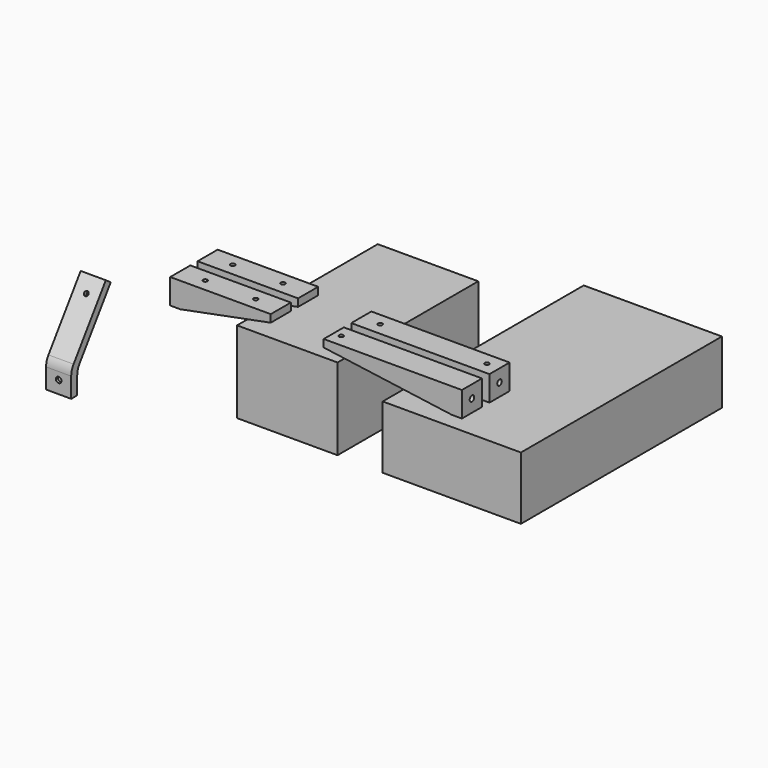
from build123d import *

# Parameters (mm, degrees)
F1_DEPTH   = 20
F3_R       = 1.75
F4_DEPTH   = 25
F5_R       = 3.5
F5_R_2     = 1.75
F6_DEPTH   = 3
F2_R       = 2.25
F7_DEPTH   = 25
F2_R_2     = 4
F8_DEPTH   = 4
F9_R       = 13
F10_W      = 80
F10_H      = 140
F11_DEPTH  = 65
F12_W      = 110
F12_H      = 200
F13_DEPTH  = 50
F15_DEPTH  = 20
F16_R      = 2.25
F17_DEPTH  = 122.8202211986
F18_DEPTH  = 4
F20_W      = 73.3484832836
F20_H      = 4
F22_R      = 1.75
F23_DEPTH  = 6.001
F22_R_2    = 3
F24_DEPTH  = 3
F26_DEPTH  = 20
F27_R      = 2.25
F28_DEPTH  = 4
F29_DEPTH  = 8.001
F31_W      = 102.9563014099
F31_H      = 4
F34_R      = 3
F34_R_2    = 1.75
F35_R      = 3
F35_R_2    = 1.75
F36_DEPTH  = 3
F36_FACE_R = 1.75
F37_DEPTH  = 9.6879868636
F38_DEPTH  = 3


with BuildPart() as f1:
    # F0 (on Right) → F1 (new body)
    with BuildSketch(Plane.YZ):
        Polygon((0, 20), (0, 0), (6, 0), (6, 18.1082072667), (39.3294984468, 65.7076640392), (34.4145861811, 69.1491226573), align=None)
    extrude(amount=F1_DEPTH)

    # F3 (on face) → F4 (cut)
    with BuildSketch(Plane(origin=(0, -9.3969262079, 6.5797985667), x_dir=(1, 0, 0), z_dir=(0, -0.8191520443, 0.5735764364))):
        with Locations((10, 64.3830408858)):
            Circle(F3_R)
    extrude(amount=-F4_DEPTH, mode=Mode.SUBTRACT)

    # F5 (on face) → F6 (cut)
    with BuildSketch(Plane(origin=(0, -4.4820139421, 3.1383399486), x_dir=(-1, 0, 0), z_dir=(0, 0.8191520443, -0.5735764364))):
        with Locations((-10, 64.3830408858)):
            Circle(F5_R)
        with Locations((-10, 64.3830408858)):
            Circle(F5_R_2, mode=Mode.SUBTRACT)
    extrude(amount=-F6_DEPTH, mode=Mode.SUBTRACT)

    # F2 (on face) → F7 (cut)
    with BuildSketch(Plane(origin=(0, 6, 0), x_dir=(-1, 0, 0), z_dir=(0, 1, 0))):
        with Locations((-10, 10)):
            Circle(F2_R)
    extrude(amount=-F7_DEPTH, mode=Mode.SUBTRACT)

    # F2 (on face) → F8 (cut)
    with BuildSketch(Plane(origin=(0, 6, 0), x_dir=(-1, 0, 0), z_dir=(0, 1, 0))):
        with Locations((-10, 10)):
            Circle(F2_R_2)
        with Locations((-10, 10)):
            Circle(F2_R, mode=Mode.SUBTRACT)
    extrude(amount=-F8_DEPTH, mode=Mode.SUBTRACT)

    # F9
    f9_edges = [f1.edges().sort_by_distance(p)[0] for p in [
        (10, 6, 18.108207),
        (10, 0, 20),
    ]]
    fillet(f9_edges, radius=F9_R)


with BuildPart() as f11:
    # F10 (on Top) → F11 (new body)
    with BuildSketch(Plane.XY):
        with Locations((156.6803222895, 114.1342443228)):
            Rectangle(F10_W, F10_H)
    extrude(amount=F11_DEPTH)


with BuildPart() as f13:
    # F12 (on Top) → F13 (new body)
    with BuildSketch(Plane.XY):
        with Locations((288.3580553532, 143.2215481997)):
            Rectangle(F12_W, F12_H)
    extrude(amount=F13_DEPTH)


with BuildPart() as f15:
    # F14 (on Front) → F15 (new body)
    with BuildSketch(Plane.XZ):
        Polygon((114.8192211986, 124.3457761407), (114.8192211986, 104.3457761407), (122.8192211986, 104.3457761407), (122.8192211986, 118.3457761407), (194.8192211986, 118.3457761407), (194.8192211986, 124.3457761407), align=None)
    extrude(amount=F15_DEPTH)

    # F16 (on face) → F17 (cut, through all)
    with BuildSketch(Plane.YZ.offset(122.8192211986)):
        with Locations((-10, 114.3457761407)):
            Circle(F16_R)
    extrude(amount=-F17_DEPTH, mode=Mode.SUBTRACT)

    # F16 (on face) → F18 (cut)
    with BuildSketch(Plane.YZ.offset(122.8192211986)):
        with BuildLine():
            ThreePointArc((-10, 118.3457761407), (-12.8284271247, 111.5173490159), (-6, 114.3457761407))
            ThreePointArc((-6, 114.3457761407), (-7.1715728753, 117.1742032654), (-10, 118.3457761407))
        make_face()
        with Locations((-10, 114.3457761407)):
            Circle(F16_R, mode=Mode.SUBTRACT)
    extrude(amount=-F18_DEPTH, mode=Mode.SUBTRACT)

    # F20 (on 3pt) → F21 (join, up to the next surface of F15)
    with BuildSketch(Plane(origin=(-15.0758317834, 0, 77.532849172), x_dir=(0.9816153897, 0, 0.1908696591), z_dir=(-0.1908696591, 0, 0.9816153897))):
        with Locations((177.1519220381, -18)):
            Rectangle(F20_W, F20_H)
        with Locations((177.1519220381, -2)):
            Rectangle(F20_W, F20_H)
    extrude(until=Until.NEXT)

    # F22 (on face) → F23 (cut, through all)
    with BuildSketch(Plane(origin=(0, 0, 118.3457761407), x_dir=(1, 0, 0), z_dir=(0, 0, -1))):
        with Locations((134.8192211986, 10)):
            Circle(F22_R)
        with Locations((174.8192211986, 10)):
            Circle(F22_R)
    extrude(amount=-F23_DEPTH, mode=Mode.SUBTRACT)

    # F22 (on face) → F24 (cut)
    with BuildSketch(Plane(origin=(0, 0, 118.3457761407), x_dir=(1, 0, 0), z_dir=(0, 0, -1))):
        with Locations((134.8192211986, 10)):
            Circle(F22_R_2)
        with Locations((134.8192211986, 10)):
            Circle(F22_R, mode=Mode.SUBTRACT)
        with Locations((174.8192211986, 10)):
            Circle(F22_R_2)
        with Locations((174.8192211986, 10)):
            Circle(F22_R, mode=Mode.SUBTRACT)
    extrude(amount=-F24_DEPTH, mode=Mode.SUBTRACT)


with BuildPart() as f26:
    # F25 (on Front) → F26 (new body)
    with BuildSketch(Plane.XZ):
        Polygon((338.9809150696, 114.6587892771), (338.9809150696, 100.6587892771), (346.9809150696, 100.6587892771), (346.9809150696, 120.6587892771), (236.9809150696, 120.6587892771), (236.9809150696, 114.6587892771), align=None)
    extrude(amount=F26_DEPTH)

    # F27 (on face) → F28 (cut)
    with BuildSketch(Plane(origin=(338.9809150696, 0, 0), x_dir=(0, -1, 0), z_dir=(-1, 0, 0))):
        with BuildLine():
            ThreePointArc((10, 114.6587892771), (7.1715728753, 107.8303621523), (14, 110.6587892771))
            ThreePointArc((14, 110.6587892771), (12.8284271247, 113.4872164018), (10, 114.6587892771))
        make_face()
        with Locations((10, 110.6587892771)):
            Circle(F27_R, mode=Mode.SUBTRACT)
    extrude(amount=-F28_DEPTH, mode=Mode.SUBTRACT)

    # F29 (cut, through all): a face of the model
    f29_faces = [f26.faces().sort_by_distance(p)[0] for p in [
        (338.9809150696, -10, 110.6587892771),
    ]]
    extrude(f29_faces, amount=-F29_DEPTH, mode=Mode.SUBTRACT)

    # F31 (on 3pt) → F32 (join, up to the next surface of F26)
    with BuildSketch(Plane(origin=(19.8283972114, 0, 144.4640368262), x_dir=(0.9907115796, 0, -0.1359800207), z_dir=(0.1359800207, 0, 0.9907115796))):
        with Locations((270.6665828668, -18)):
            Rectangle(F31_W, F31_H)
        with Locations((270.6665828668, -2)):
            Rectangle(F31_W, F31_H)
    extrude(until=Until.NEXT)


with BuildPart() as f33_1:
    # F33: copy of F26
    add(f26.part.moved(Location((0, 27.4, 0))))


with BuildPart() as f36_tool:
    # F34 (on face) + F35 (on face) → F36 (new body)
    with BuildSketch(Plane(origin=(0, 0, 114.6587892771), x_dir=(1, 0, 0), z_dir=(0, 0, -1))):
        with Locations((242.9809150696, 10)):
            Circle(F34_R)
        with Locations((242.9809150696, 10)):
            Circle(F34_R_2, mode=Mode.SUBTRACT)
    with BuildSketch(Plane(origin=(0, 0, 114.6587892771), x_dir=(1, 0, 0), z_dir=(0, 0, -1))):
        with Locations((251.9809150696, -17.4)):
            Circle(F35_R)
        with Locations((251.9809150696, -17.4)):
            Circle(F35_R_2, mode=Mode.SUBTRACT)
        with BuildLine():
            Line((338.9809150696, -17.4), (338.9809150696, -15.1639320225))
            ThreePointArc((338.9809150696, -15.1639320225), (333.9809150696, -17.4), (338.9809150696, -19.6360679775))
            Line((338.9809150696, -19.6360679775), (338.9809150696, -17.4))
        make_face()
        with Locations((336.9809150696, -17.4)):
            Circle(F35_R_2, mode=Mode.SUBTRACT)
    extrude(amount=-F36_DEPTH)


with BuildPart() as f26_1:
    add(f26.part)

    # F36: cut by f36_tool
    add(f36_tool.part, mode=Mode.SUBTRACT)


with BuildPart() as f33_1_1:
    add(f33_1.part)

    # F36: cut by f36_tool
    add(f36_tool.part, mode=Mode.SUBTRACT)


with BuildPart() as f37_tool:
    # F36_face (on face) → F37 (new body, through all)
    with BuildSketch(Plane(origin=(242.9809150696, -10, 114.6587892771), x_dir=(1, 0, 0), z_dir=(0, 0, -1))):
        Circle(F36_FACE_R)
        with Locations((9, -27.4)):
            Circle(F36_FACE_R)
        with Locations((94, -27.4)):
            Circle(F36_FACE_R)
    extrude(amount=-F37_DEPTH)


with BuildPart() as f26_2:
    add(f26_1.part)

    # F37: cut by f37_tool
    add(f37_tool.part, mode=Mode.SUBTRACT)


with BuildPart() as f33_1_2:
    add(f33_1_1.part)

    # F37: cut by f37_tool
    add(f37_tool.part, mode=Mode.SUBTRACT)

    # F35 (on face) → F38 (cut, symmetric)
    with BuildSketch(Plane(origin=(0, 0, 114.6587892771), x_dir=(1, 0, 0), z_dir=(0, 0, -1))):
        with BuildLine():
            ThreePointArc((338.9809150696, -19.6360679775), (339.7195278571, -18.6247448714), (339.9809150696, -17.4))
            ThreePointArc((339.9809150696, -17.4), (339.7195278571, -16.1752551286), (338.9809150696, -15.1639320225))
            Line((338.9809150696, -15.1639320225), (338.9809150696, -17.4))
            Line((338.9809150696, -17.4), (338.9809150696, -19.6360679775))
        make_face()
    extrude(amount=F38_DEPTH, both=True, mode=Mode.SUBTRACT)


with BuildPart() as f39_1:
    # F39: copy of F15
    add(f15.part.moved(Location((0, 27.2, 0))))


solid = Compound([f1.part, f11.part, f13.part, f15.part, f26_2.part, f33_1_2.part, f39_1.part])
